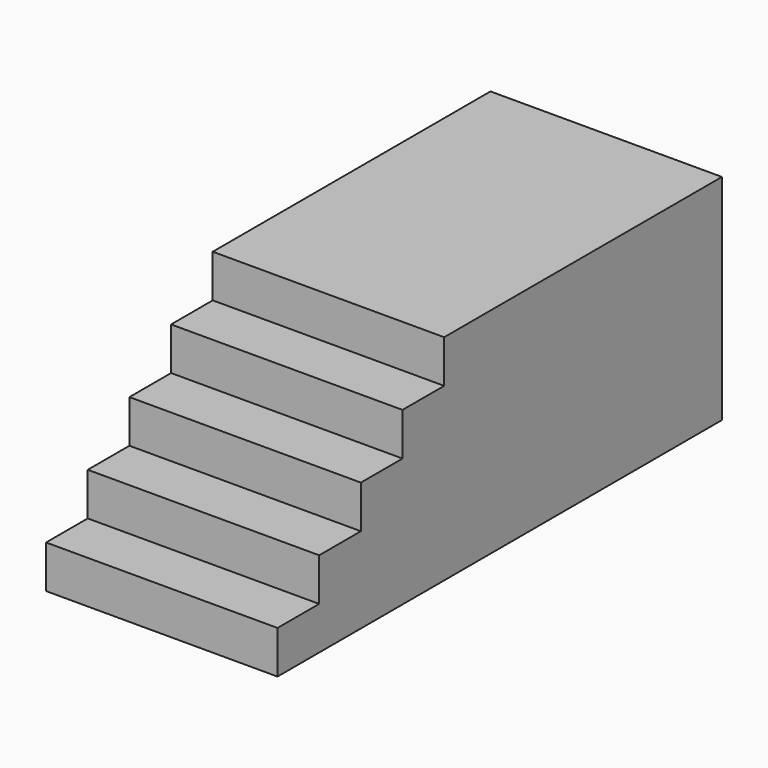
from build123d import *

# Parameters (mm, degrees)
F0_W      = 4876.8
F0_H      = 1066.8
F1_DEPTH  = 101.6
F3_DEPTH  = 1016
F7_W      = 3860.8
F7_H      = 1066.8
F8_DEPTH  = 458.42061
F9_W      = 1016
F9_H      = 939.8
F10_DEPTH = 457.2


# Not quite as in the source:
# - a feature of the source that left no trace in its solid (it failed there, or was rolled back) is left out


with BuildPart() as f1:
    # F0 (on Top) → F1 (new body)
    with BuildSketch(Plane.XY):
        Rectangle(F0_W, F0_H)
    extrude(amount=-F1_DEPTH)

    # F2 (on face) → F3 (join)
    with BuildSketch(Plane(origin=(-2438.4, 0, 0), x_dir=(0, -1, 0), z_dir=(-1, 0, 0))):
        Polygon((533.4, -187.96), (533.4, 0), (304.8, 0), (-533.4, 0), (-533.4, -939.8), (304.8, -939.8), (1447.8, -939.8), (1447.8, -751.84), (1219.2, -751.84), (1219.2, -563.88), (990.6, -563.88), (990.6, -375.92), (762, -375.92), (762, -187.96), align=None)
    extrude(amount=-F3_DEPTH)

    # F7 (on face) → F8 (cut)
    with BuildSketch(Plane.XY):
        with Locations((508, 0)):
            Rectangle(F7_W, F7_H)
    extrude(amount=-F8_DEPTH, mode=Mode.SUBTRACT)

    # F9 (on face) → F10 (join)
    with BuildSketch(Plane(origin=(0, 533.4, 0), x_dir=(-1, 0, 0), z_dir=(0, 1, 0))):
        with Locations((1930.4, -469.9)):
            Rectangle(F9_W, F9_H)
    extrude(amount=F10_DEPTH)


solid = f1.part
